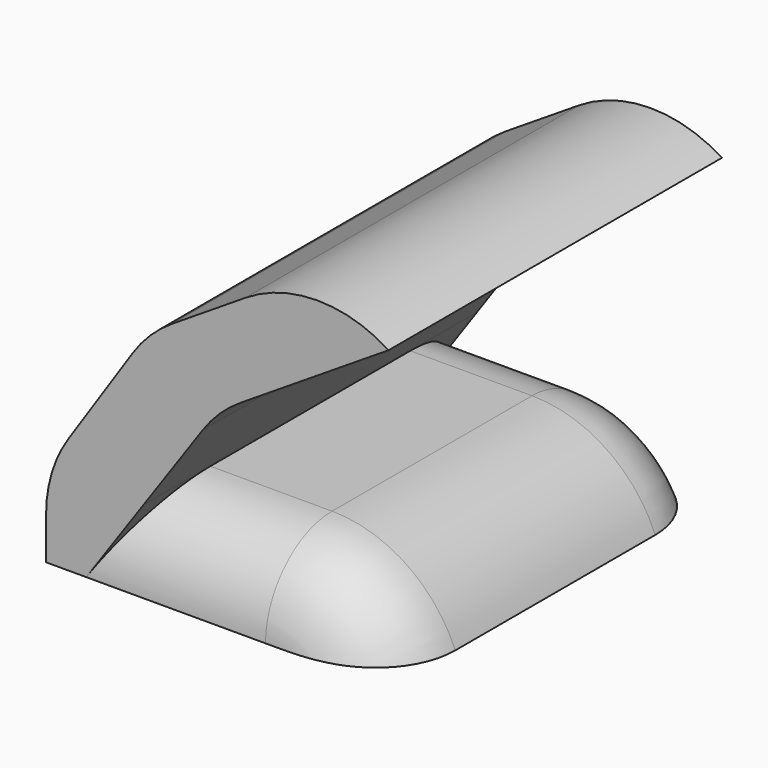
from build123d import *

# Parameters (mm, degrees)
F1_DEPTH     = 12.5
F2_T1_DEPTH  = 75.8666564448
F2_T3_DEPTH  = 33.4238697913
F2_T5_DEPTH  = 37.1110249992
F2_T7_DEPTH  = 61.9747717196
F3_T2_ANGLE  = 157.1183672373
F3_T4_ANGLE  = 157.1183672373
F3_T8_DEPTH  = 19.8096921988
F3_T13_DEPTH = 19.8096921988
F4_R         = 8


# Not quite as in the source:
# - a fillet or chamfer that OpenCascade refuses, or shapes differently, is made with other operations: its cross-section is extruded or revolved along the edge and cut away or added


with BuildPart() as f1:
    # F0 (on Front) → F1 (new body, symmetric)
    with BuildSketch(Plane.XZ):
        Polygon((-20.558629185, 0), (0, 0), (0, 4.9480088055), (-14.7046465427, 4.9480088055), (-10.2444691584, 11.3595137373), (0, 17.8922185832), (0, 23.3462397009), (-14.4258858636, 14.1471242532), (-20.558629185, 4.9480088055), align=None)
    extrude(amount=F1_DEPTH, both=True)

    # F2: fillet of radius 8 on 4 edges, made by hand

    # F2_s2 → F2_t1 (cut)
    with BuildSketch(Plane.XZ.offset(-37.9333282224)):
        with BuildLine():
            ThreePointArc((-8.5777252412, 17.8763860282), (-4.2911639454, 19.1311087323), (0, 17.8922185832))
            Line((0, 17.8922185832), (0, 23.3462397009))
            Line((0, 23.3462397009), (-8.5777252412, 17.8763860282))
        make_face()
    extrude(amount=F2_T1_DEPTH, mode=Mode.SUBTRACT)

    # F2_s4 → F2_t3 (cut)
    with BuildSketch(Plane.XZ.offset(-16.7119348957)):
        with BuildLine():
            ThreePointArc((-15.3604302761, 12.7453075635), (-14.3030712709, 14.0217863385), (-13.0053552923, 15.0529698176))
            Line((-13.0053552923, 15.0529698176), (-14.4258858636, 14.1471242532))
            Line((-14.4258858636, 14.1471242532), (-15.3604302761, 12.7453075635))
        make_face()
    extrude(amount=F2_T3_DEPTH, mode=Mode.SUBTRACT)

    # F2_s6 → F2_t5 (cut)
    with BuildSketch(Plane.XZ.offset(-18.5555124996)):
        with BuildLine():
            ThreePointArc((-20.558629185, 2.5258038057), (-20.215365424, 4.8440769057), (-19.2150316433, 6.96340522))
            Line((-19.2150316433, 6.96340522), (-20.558629185, 4.9480088055))
            Line((-20.558629185, 4.9480088055), (-20.558629185, 2.5258038057))
        make_face()
    extrude(amount=F2_T5_DEPTH, mode=Mode.SUBTRACT)

    # F2_s8 → F2_t7 (cut)
    with BuildSketch(Plane.XZ.offset(-30.9873858598)):
        with BuildLine():
            ThreePointArc((-7.3949543439, 4.9480088055), (-2.9461303171, 3.5969158419), (0, 0))
            Line((0, 0), (0, 4.9480088055))
            Line((0, 4.9480088055), (-7.3949543439, 4.9480088055))
        make_face()
    extrude(amount=F2_T7_DEPTH, mode=Mode.SUBTRACT)

    # F3: fillet of radius 5 on 4 edges, made by hand

    # F3_s1 → F3_t2 (revolve, cut)
    with BuildSketch(Plane.YZ.offset(-7.3949543439)):
        with BuildLine():
            ThreePointArc((12.5, -0.0519911945), (11.0355339059, 3.4835427114), (7.5, 4.9480088055))
            Line((7.5, 4.9480088055), (12.5, 4.9480088055))
            Line((12.5, 4.9480088055), (12.5, -0.0519911945))
        make_face()
    revolve(axis=Axis((-7.3949543439, 12.5, -3.0519911944), (0, 1, 0)), revolution_arc=F3_T2_ANGLE, mode=Mode.SUBTRACT)

    # F3_s3 → F3_t4 (revolve, cut)
    with BuildSketch(Plane.YZ.offset(-7.3949543439)):
        with BuildLine():
            ThreePointArc((-12.5, -0.0519911945), (-11.0355339059, 3.4835427114), (-7.5, 4.9480088055))
            Line((-7.5, 4.9480088055), (-12.5, 4.9480088055))
            Line((-12.5, 4.9480088055), (-12.5, -0.0519911945))
        make_face()
    revolve(axis=Axis((-7.3949543439, -12.5, -3.0519911944), (0, 1, 0)), revolution_arc=F3_T4_ANGLE, mode=Mode.SUBTRACT)


with BuildPart() as f3_tool6:
    # F3_s7 → F3_t8 (new body)
    with BuildSketch(Plane.YZ.offset(-7.3949543439)):
        with BuildLine():
            ThreePointArc((-12.5, -0.0519911945), (-11.0355339059, 3.4835427114), (-7.5, 4.9480088055))
            Line((-7.5, 4.9480088055), (-12.5, 4.9480088055))
            Line((-12.5, 4.9480088055), (-12.5, -0.0519911945))
        make_face()
    extrude(amount=-F3_T8_DEPTH)

    split(bisect_by=Plane(origin=(-12.2288219378, 0, 8.5070066427), x_dir=(0, 1, 0), z_dir=(0.8209051994, 0, -0.5710644917)), keep=Keep.TOP)


with BuildPart() as f1_1:
    add(f1.part)

    # F3_t5: cut F3_tool6
    add(f3_tool6.part, mode=Mode.SUBTRACT)


with BuildPart() as f3_tool11:
    # F3_s12 → F3_t13 (new body)
    with BuildSketch(Plane.YZ.offset(-7.3949543439)):
        with BuildLine():
            ThreePointArc((12.5, -0.0519911945), (11.0355339059, 3.4835427114), (7.5, 4.9480088055))
            Line((7.5, 4.9480088055), (12.5, 4.9480088055))
            Line((12.5, 4.9480088055), (12.5, -0.0519911945))
        make_face()
    extrude(amount=-F3_T13_DEPTH)

    split(bisect_by=Plane(origin=(-12.2288219378, 0, 8.5070066427), x_dir=(0, 1, 0), z_dir=(0.8209051994, 0, -0.5710644917)), keep=Keep.TOP)


with BuildPart() as f1_2:
    add(f1_1.part)

    # F3_t10: cut F3_tool11
    add(f3_tool11.part, mode=Mode.SUBTRACT)

    # F4
    f4_edges = [f1_2.edges().sort_by_distance(p)[0] for p in [
        (-10.244469, 0, 11.359514),
    ]]
    fillet(f4_edges, radius=F4_R)


solid = f1_2.part
